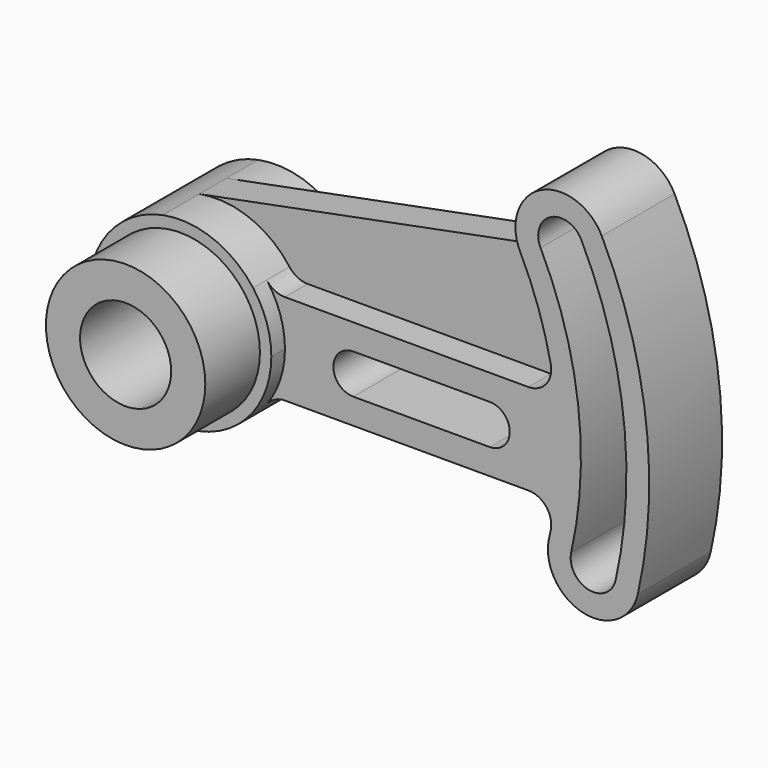
from build123d import *
from build123d import SkipClean  # not in build123d's __all__

# Parameters (mm, degrees)
F0_R     = 22.225
F1_DEPTH = 33.3248
F0_R_2   = 12.7
F2_DEPTH = 52.3748
F3_DEPTH = 28.575
F4_DEPTH = 20.6248
F5_DEPTH = 3.175
F6_DEPTH = 11.0998
F7_ANGLE = 90


with BuildPart() as f1:
    # F0 (on Top) → F1 (new body)
    with BuildSketch(Plane.XY):
        with BuildLine():
            ThreePointArc((20.32, 15.24), (9.1294627068, 23.7025929106), (-4.8465484826, 24.9333304596))
            ThreePointArc((-4.8465484826, 24.9333304596), (-21.5251259118, -13.4843967044), (20.32, -15.24))
            ThreePointArc((20.32, -15.24), (24.0965557705, -8.0321852568), (25.4, 0))
            ThreePointArc((25.4, 0), (24.0965557705, 8.0321852568), (20.32, 15.24))
        make_face()
        Circle(F0_R, mode=Mode.SUBTRACT)
    extrude(amount=F1_DEPTH)

    # F0 (on Top) → F2 (join)
    with BuildSketch(Plane.XY):
        Circle(F0_R)
        Circle(F0_R_2, mode=Mode.SUBTRACT)
    extrude(amount=F2_DEPTH)

    # F0 (on Top) → F3 (join)
    with BuildSketch(Plane.XY):
        with BuildLine():
            ThreePointArc((123.8244974665, -28.2222222222), (126.1134026015, 14.9803098855), (113.7674148927, 56.4444444444))
            ThreePointArc((113.7674148927, 56.4444444444), (98.7718041015, 62.9734869687), (89.7780268905, 49.313007081))
            ThreePointArc((89.7780268905, 49.313007081), (90.2171864347, 47.1811306981), (91.0139319141, 45.1555555556))
            ThreePointArc((91.0139319141, 45.1555555556), (96.0863854596, 33.0146411355), (99.5472631467, 20.32))
            ThreePointArc((99.5472631467, 20.32), (98.2442480497, 15.0339073716), (93.3255592, 12.7))
            Line((93.3255592, 12.7), (57.15, 12.7))
            Line((57.15, 12.7), (25.4, 12.7))
            ThreePointArc((25.4, 12.7), (22.5601936686, 13.3703873372), (20.32, 15.24))
            ThreePointArc((20.32, 15.24), (24.0965557705, 8.0321852568), (25.4, 0))
            ThreePointArc((25.4, 0), (24.0965557705, -8.0321852568), (20.32, -15.24))
            ThreePointArc((20.32, -15.24), (22.5601936686, -13.3703873372), (25.4, -12.7))
            Line((25.4, -12.7), (54.6792037785, -12.7))
            Line((54.6792037785, -12.7), (93.3255592, -12.7))
            ThreePointArc((93.3255592, -12.7), (98.2442480497, -15.0339073716), (99.5472631467, -20.32))
            ThreePointArc((99.5472631467, -20.32), (99.3098469997, -21.4502747977), (99.0595979732, -22.5777777778))
            ThreePointArc((99.0595979732, -22.5777777778), (108.6198254977, -37.7824497467), (123.8244974665, -28.2222222222))
        make_face()
        with BuildLine():
            ThreePointArc((82.55, 5.5499), (88.0999, 0), (82.55, -5.5499))
            Line((82.55, -5.5499), (44.45, -5.5499))
            ThreePointArc((44.45, -5.5499), (38.9001, 0), (44.45, 5.5499))
            Line((44.45, 5.5499), (82.55, 5.5499))
        make_face(mode=Mode.SUBTRACT)
        with BuildLine():
            ThreePointArc((117.6332725932, -26.8111111111), (110.0309366088, -31.5912248733), (105.2508228466, -23.9888888889))
            ThreePointArc((105.2508228466, -23.9888888889), (107.1963922113, 12.7332634026), (96.7023026588, 47.9777777778))
            ThreePointArc((96.7023026588, 47.9777777778), (99.5684511812, 56.4883707446), (108.079044148, 53.6222222222))
            ThreePointArc((108.079044148, 53.6222222222), (119.8077324715, 14.2312943912), (117.6332725932, -26.8111111111))
        make_face(mode=Mode.SUBTRACT)
    extrude(amount=F3_DEPTH)

    # F0 (on Top) → F4 (join)
    with BuildSketch(Plane.XY):
        with BuildLine():
            ThreePointArc((91.0139319141, 45.1555555556), (90.2171864347, 47.1811306981), (89.7780268905, 49.313007081))
            ThreePointArc((89.7780268905, 49.313007081), (88.599955582, 44.8247099647), (84.6833407547, 42.3361780066))
            Line((84.6833407547, 42.3361780066), (-4.8465484826, 24.9333304596))
            ThreePointArc((-4.8465484826, 24.9333304596), (9.1294627068, 23.7025929106), (20.32, 15.24))
            ThreePointArc((20.32, 15.24), (22.5601936686, 13.3703873372), (25.4, 12.7))
            Line((25.4, 12.7), (57.15, 12.7))
            Line((57.15, 12.7), (93.3255592, 12.7))
            ThreePointArc((93.3255592, 12.7), (98.2442480497, 15.0339073716), (99.5472631467, 20.32))
            ThreePointArc((99.5472631467, 20.32), (96.0863854596, 33.0146411355), (91.0139319141, 45.1555555556))
        make_face()
    extrude(amount=F4_DEPTH)

    # F0 (on Top) → F5 (cut)
    with BuildSketch(Plane.XY):
        with BuildLine():
            ThreePointArc((123.8244974665, -28.2222222222), (126.1134026015, 14.9803098855), (113.7674148927, 56.4444444444))
            ThreePointArc((113.7674148927, 56.4444444444), (98.7718041015, 62.9734869687), (89.7780268905, 49.313007081))
            ThreePointArc((89.7780268905, 49.313007081), (90.2171864347, 47.1811306981), (91.0139319141, 45.1555555556))
            ThreePointArc((91.0139319141, 45.1555555556), (96.0863854596, 33.0146411355), (99.5472631467, 20.32))
            ThreePointArc((99.5472631467, 20.32), (98.2442480497, 15.0339073716), (93.3255592, 12.7))
            Line((93.3255592, 12.7), (57.15, 12.7))
            Line((57.15, 12.7), (25.4, 12.7))
            ThreePointArc((25.4, 12.7), (22.5601936686, 13.3703873372), (20.32, 15.24))
            ThreePointArc((20.32, 15.24), (24.0965557705, 8.0321852568), (25.4, 0))
            ThreePointArc((25.4, 0), (24.0965557705, -8.0321852568), (20.32, -15.24))
            ThreePointArc((20.32, -15.24), (22.5601936686, -13.3703873372), (25.4, -12.7))
            Line((25.4, -12.7), (54.6792037785, -12.7))
            Line((54.6792037785, -12.7), (93.3255592, -12.7))
            ThreePointArc((93.3255592, -12.7), (98.2442480497, -15.0339073716), (99.5472631467, -20.32))
            ThreePointArc((99.5472631467, -20.32), (99.3098469997, -21.4502747977), (99.0595979732, -22.5777777778))
            ThreePointArc((99.0595979732, -22.5777777778), (108.6198254977, -37.7824497467), (123.8244974665, -28.2222222222))
        make_face()
        with BuildLine():
            ThreePointArc((82.55, 5.5499), (88.0999, 0), (82.55, -5.5499))
            Line((82.55, -5.5499), (44.45, -5.5499))
            ThreePointArc((44.45, -5.5499), (38.9001, 0), (44.45, 5.5499))
            Line((44.45, 5.5499), (82.55, 5.5499))
        make_face(mode=Mode.SUBTRACT)
        with BuildLine():
            ThreePointArc((117.6332725932, -26.8111111111), (110.0309366088, -31.5912248733), (105.2508228466, -23.9888888889))
            ThreePointArc((105.2508228466, -23.9888888889), (107.1963922113, 12.7332634026), (96.7023026588, 47.9777777778))
            ThreePointArc((96.7023026588, 47.9777777778), (99.5684511812, 56.4883707446), (108.079044148, 53.6222222222))
            ThreePointArc((108.079044148, 53.6222222222), (119.8077324715, 14.2312943912), (117.6332725932, -26.8111111111))
        make_face(mode=Mode.SUBTRACT)
    with SkipClean():  # cleaning this boolean's faces spoils the solid; the shape is the same uncleaned
        extrude(amount=F5_DEPTH, mode=Mode.SUBTRACT)

    # F0 (on Top) → F6 (cut)
    with BuildSketch(Plane.XY):
        with BuildLine():
            ThreePointArc((91.0139319141, 45.1555555556), (90.2171864347, 47.1811306981), (89.7780268905, 49.313007081))
            ThreePointArc((89.7780268905, 49.313007081), (88.599955582, 44.8247099647), (84.6833407547, 42.3361780066))
            Line((84.6833407547, 42.3361780066), (-4.8465484826, 24.9333304596))
            ThreePointArc((-4.8465484826, 24.9333304596), (9.1294627068, 23.7025929106), (20.32, 15.24))
            ThreePointArc((20.32, 15.24), (22.5601936686, 13.3703873372), (25.4, 12.7))
            Line((25.4, 12.7), (57.15, 12.7))
            Line((57.15, 12.7), (93.3255592, 12.7))
            ThreePointArc((93.3255592, 12.7), (98.2442480497, 15.0339073716), (99.5472631467, 20.32))
            ThreePointArc((99.5472631467, 20.32), (96.0863854596, 33.0146411355), (91.0139319141, 45.1555555556))
        make_face()
    with SkipClean():  # cleaning this boolean's faces spoils the solid; the shape is the same uncleaned
        extrude(amount=F6_DEPTH, mode=Mode.SUBTRACT)


with BuildPart() as f1_1:
    # F7: moved
    add(f1.part.rotate(Axis((59.3627796, 12.7, 28.575), (1, 0, 0)), F7_ANGLE), clean=False)


solid = f1_1.part
